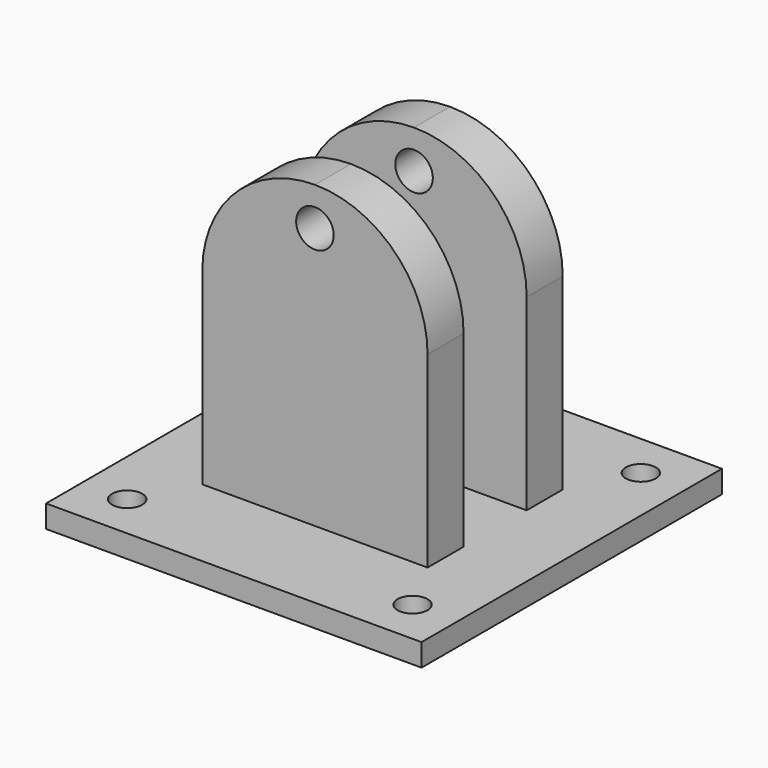
from build123d import *

# Parameters (mm, degrees)
F0_W      = 50
F0_H      = 50
F1_DEPTH  = 3
F2_W      = 30
F2_H      = 6
F3_DEPTH  = 40
F4_W      = 30
F4_H      = 6
F5_DEPTH  = 40
F6_R      = 14.99999
F7_R      = 14.99999
F9_D      = 5
F12_D     = 4
F12_DEPTH = 15
F12_TIP   = 1.2017212381


# Not quite as in the source:
# - a fillet or chamfer is up to 0.001 mm smaller than in the source, because OpenCascade refuses the exact size


with BuildPart() as f1:
    # F0 (on Top) → F1 (new body)
    with BuildSketch(Plane.XY):
        with Locations((1.1680303141, 2.4703653681)):
            Rectangle(F0_W, F0_H)
    extrude(amount=F1_DEPTH)

    # F2 (on face) → F3 (join)
    with BuildSketch(Plane.XY.offset(3)):
        with Locations((1.1680303141, -6.0296346319)):
            Rectangle(F2_W, F2_H)
    extrude(amount=F3_DEPTH)

    # F4 (on face) → F5 (join)
    with BuildSketch(Plane.XY.offset(3)):
        with Locations((1.1680303141, 10.4703653681)):
            Rectangle(F4_W, F4_H)
    extrude(amount=F5_DEPTH)

    # F6 (radius 15 in the source; OpenCascade refuses exactly that, so slightly less here)
    f6_edges = [f1.edges().sort_by_distance(p)[0] for p in [
        (-13.83197, -6.029635, 43),
        (16.16803, -6.029635, 43),
    ]]
    fillet(f6_edges, radius=F6_R)

    # F7 (radius 15 in the source; OpenCascade refuses exactly that, so slightly less here)
    f7_edges = [f1.edges().sort_by_distance(p)[0] for p in [
        (16.16803, 10.470365, 43),
        (-13.83197, 10.470365, 43),
    ]]
    fillet(f7_edges, radius=F7_R)

    # F9 (through all)
    with Locations(Plane.XZ.offset(9.0296346319)):
        with Locations((1.1680303141, 37.8934629261)):
            Hole(F9_D / 2)

    # F12
    with Locations(Plane.XY.offset(3)):
        with Locations((-17.8319696859, 21.4703653681), (20.1680303141, 21.4703653681), (20.1680303141, -16.5296346319), (-17.8319696859, -16.5296346319)):
            Hole(F12_D / 2, depth=F12_DEPTH)
            with Locations((0, 0, -(F12_DEPTH + F12_TIP / 2))):  # 118° drill point
                Cone(0, F12_D / 2, F12_TIP, mode=Mode.SUBTRACT)


solid = f1.part
